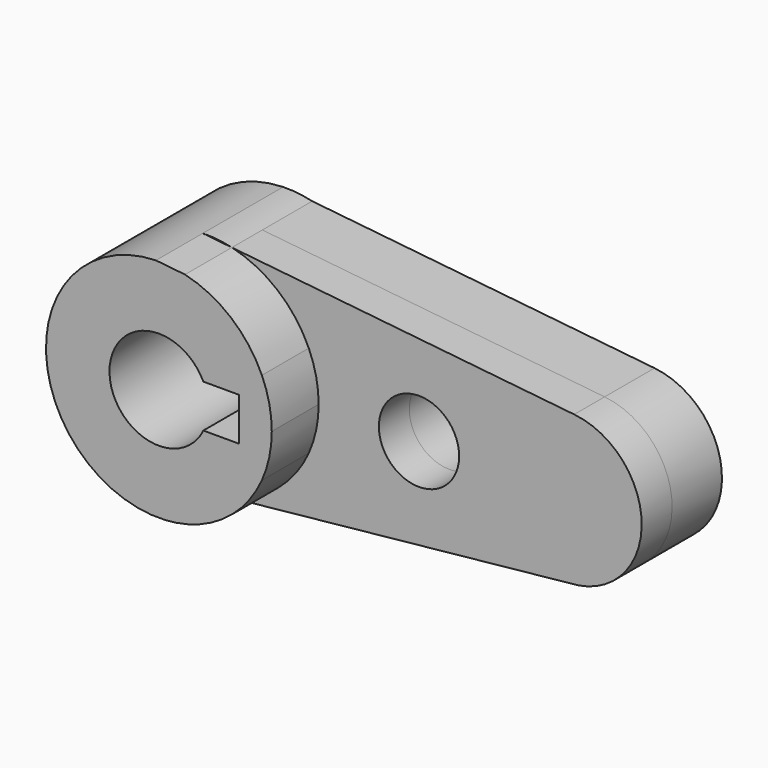
from build123d import *

# Parameters (mm, degrees)
F0_R     = 25.920114285
F0_R_2   = 10.16
F1_DEPTH = 25.4
F2_DEPTH = 40.2336
F3_DEPTH = 15.7734


with BuildPart() as f1:
    # F0 (on Front) → F1 (new body)
    with BuildSketch(Plane.XZ):
        with BuildLine():
            Line((-59.5011196988, 27.7984474733), (-66.8666748677, 28.5651783385))
            ThreePointArc((-66.8666748677, 28.5651783385), (-94.6693896394, -1.1498632737), (-64.5671747022, -28.532910996))
            Line((-64.5671747022, -28.532910996), (-61.8152346636, -28.2492626852))
            ThreePointArc((-61.8152346636, -28.2492626852), (-48.8211255332, -22.7456559902), (-40.0452872532, -11.6948089082))
            ThreePointArc((-40.0452872532, -11.6948089082), (-38.1752269621, -5.9798061717), (-37.5425343677, 0))
            ThreePointArc((-37.5425343677, 0), (-38.1752269621, 5.9798061717), (-40.0452872532, 11.6948089082))
            ThreePointArc((-40.0452872532, 11.6948089082), (-47.8975193826, 22.0127617291), (-59.5011196988, 27.7984474733))
        make_face()
        with Locations((-66.1175343677, 0)):
            Circle(F0_R, mode=Mode.SUBTRACT)
        with BuildLine():
            ThreePointArc((-59.5011196988, 27.7984474733), (-63.1589543708, 28.4214255343), (-66.8666748677, 28.5651783385))
            Line((-66.8666748677, 28.5651783385), (-59.5011196988, 27.7984474733))
        make_face()
        with BuildLine():
            Line((-61.8152346636, -28.2492626852), (-64.5671747022, -28.532910996))
            ThreePointArc((-64.5671747022, -28.532910996), (-63.1877699548, -28.4244103806), (-61.8152346636, -28.2492626852))
        make_face()
        with BuildLine():
            Line((27.1393383143, 18.7794513749), (-59.5011196988, 27.7984474733))
            ThreePointArc((-59.5011196988, 27.7984474733), (-47.8975193826, 22.0127617291), (-40.0452872532, 11.6948089082))
            ThreePointArc((-40.0452872532, 11.6948089082), (-38.1752269621, 5.9798061717), (-37.5425343677, 0))
            ThreePointArc((-37.5425343677, 0), (-38.1752269621, -5.9798061717), (-40.0452872532, -11.6948089082))
            ThreePointArc((-40.0452872532, -11.6948089082), (-48.8211255332, -22.7456559902), (-61.8152346636, -28.2492626852))
            Line((-61.8152346636, -28.2492626852), (28.2660160912, -18.9643966421))
            ThreePointArc((28.2660160912, -18.9643966421), (44.208469968, 0.4002357381), (27.1393383143, 18.7794513749))
        make_face()
        with Locations((-12.1425343677, 0)):
            Circle(F0_R_2, mode=Mode.SUBTRACT)
    extrude(amount=F1_DEPTH)


with BuildPart() as f2:
    # F0 (on Front) → F2 (new body)
    with BuildSketch(Plane.XZ):
        with BuildLine():
            Line((-59.5011196988, 27.7984474733), (-66.8666748677, 28.5651783385))
            ThreePointArc((-66.8666748677, 28.5651783385), (-94.6693896394, -1.1498632737), (-64.5671747022, -28.532910996))
            Line((-64.5671747022, -28.532910996), (-61.8152346636, -28.2492626852))
            ThreePointArc((-61.8152346636, -28.2492626852), (-48.8211255332, -22.7456559902), (-40.0452872532, -11.6948089082))
            ThreePointArc((-40.0452872532, -11.6948089082), (-38.1752269621, -5.9798061717), (-37.5425343677, 0))
            ThreePointArc((-37.5425343677, 0), (-38.1752269621, 5.9798061717), (-40.0452872532, 11.6948089082))
            ThreePointArc((-40.0452872532, 11.6948089082), (-47.8975193826, 22.0127617291), (-59.5011196988, 27.7984474733))
        make_face()
        with Locations((-66.1175343677, 0)):
            Circle(F0_R, mode=Mode.SUBTRACT)
        with Locations((-66.1175343677, 0)):
            Circle(F0_R)
        with BuildLine():
            Line((-45.8052044434, 5.4486445151), (-45.8052044434, 2.0219158244))
            Line((-45.8052044434, 2.0219158244), (-45.8052044434, 0))
            Line((-45.8052044434, 0), (-45.8052044434, -5.4486445151))
            Line((-45.8052044434, -5.4486445151), (-54.862577912, -5.4486445151))
            ThreePointArc((-54.862577912, -5.4486445151), (-55.4806143724, -6.5740174083), (-56.2107898295, -7.6300841756))
            ThreePointArc((-56.2107898295, -7.6300841756), (-78.556090686, 1.2822201807), (-54.862577912, 5.4486445151))
            Line((-54.862577912, 5.4486445151), (-45.8052044434, 5.4486445151))
        make_face(mode=Mode.SUBTRACT)
    extrude(amount=F2_DEPTH)

    # F0 (on Front) → F3 (join)
    with BuildSketch(Plane.XZ):
        with BuildLine():
            Line((27.1393383143, 18.7794513749), (-59.5011196988, 27.7984474733))
            ThreePointArc((-59.5011196988, 27.7984474733), (-47.8975193826, 22.0127617291), (-40.0452872532, 11.6948089082))
            ThreePointArc((-40.0452872532, 11.6948089082), (-38.1752269621, 5.9798061717), (-37.5425343677, 0))
            ThreePointArc((-37.5425343677, 0), (-38.1752269621, -5.9798061717), (-40.0452872532, -11.6948089082))
            ThreePointArc((-40.0452872532, -11.6948089082), (-48.8211255332, -22.7456559902), (-61.8152346636, -28.2492626852))
            Line((-61.8152346636, -28.2492626852), (28.2660160912, -18.9643966421))
            ThreePointArc((28.2660160912, -18.9643966421), (44.208469968, 0.4002357381), (27.1393383143, 18.7794513749))
        make_face()
        with Locations((-12.1425343677, 0)):
            Circle(F0_R_2, mode=Mode.SUBTRACT)
    extrude(amount=F3_DEPTH)


solid = Compound([f1.part, f2.part])
